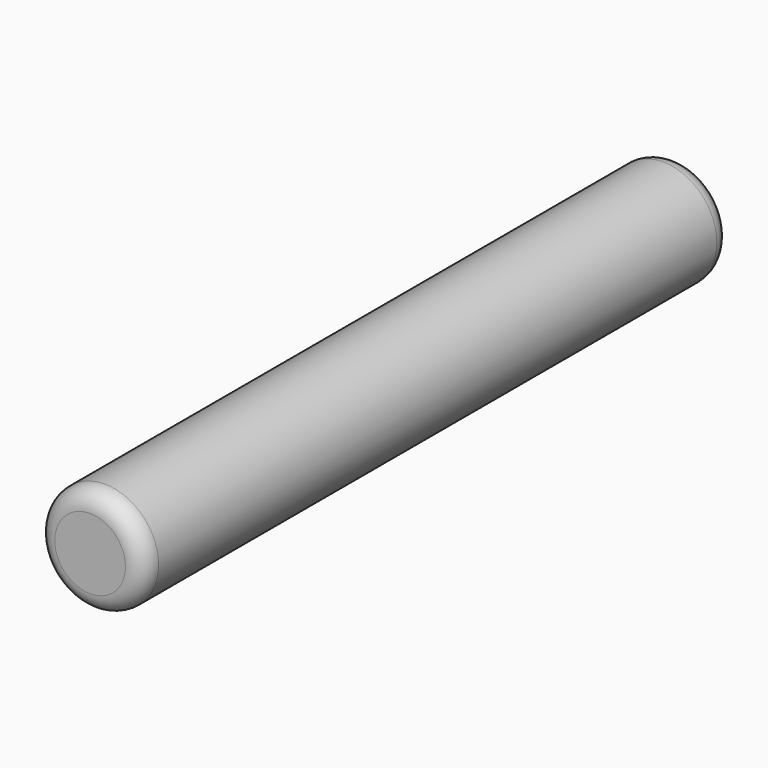
from build123d import *

# Parameters (mm, degrees)
F0_R     = 14.8623385086
F1_DEPTH = 203.2
F2_R     = 5.08


# Not quite as in the source:
# - a feature of the source that left no trace in its solid (it failed there, or was rolled back) is left out


with BuildPart() as f1:
    # F0 (on Front) → F1 (new body)
    with BuildSketch(Plane.XZ):
        Circle(F0_R)
    extrude(amount=F1_DEPTH)

    # F2
    f2_edges = [f1.edges().sort_by_distance(p)[0] for p in [
        (14.862339, -101.6, 0),
        (-14.862339, 0, 0),
        (-14.862339, -203.2, 0),
    ]]
    fillet(f2_edges, radius=F2_R)


solid = f1.part
